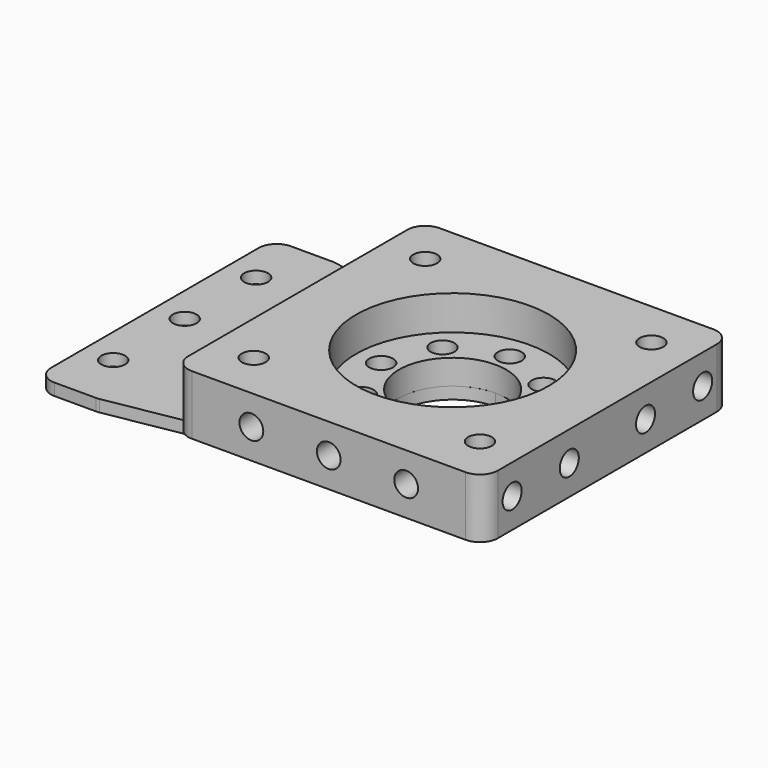
from build123d import *

# Parameters (mm, degrees)
F0_W             = 26
F0_H             = 26
F0_R             = 1
F0_R_2           = 4.5
F1_DEPTH         = 5
F2_R             = 1
F3_DEPTH         = 2
F4_R             = 8.1
F5_DEPTH         = 2.9
F6_R             = 1
F7_DEPTH         = 2
F8_R             = 1.5
F9_R             = 1
F10_DEPTH        = 5
F11_R            = 1
F12_DEPTH        = 1
F14_DEPTH        = 1
F15_R            = 1.5
F16_R            = 1
F17_DEPTH        = 4
F17_COPIES_COUNT = 2
F17_COPIES_PITCH = 22


# Not quite as in the source:
# - a pattern or mirror of a feature is missing from the dataset's text; its kind, count and spacing are read off the source's solid


with BuildPart() as f1:
    # F0 (on Top) → F1 (new body)
    with BuildSketch(Plane.XY):
        Rectangle(F0_W, F0_H)
        with Locations((-4.2426406871, -4.2426406871)):
            Circle(F0_R, mode=Mode.SUBTRACT)
        with Locations((0, -6)):
            Circle(F0_R, mode=Mode.SUBTRACT)
        with Locations((4.2426406871, -4.2426406871)):
            Circle(F0_R, mode=Mode.SUBTRACT)
        with Locations((-6, 0)):
            Circle(F0_R, mode=Mode.SUBTRACT)
        with Locations((-4.2426406871, 4.2426406871)):
            Circle(F0_R, mode=Mode.SUBTRACT)
        Circle(F0_R_2, mode=Mode.SUBTRACT)
        with Locations((6, 0)):
            Circle(F0_R, mode=Mode.SUBTRACT)
        with Locations((0, 6)):
            Circle(F0_R, mode=Mode.SUBTRACT)
        with Locations((4.2426406871, 4.2426406871)):
            Circle(F0_R, mode=Mode.SUBTRACT)
    extrude(amount=F1_DEPTH)

    # F2 (on face) → F3 (cut)
    with BuildSketch(Plane.XZ.offset(13)):
        with Locations((0, 2.5)):
            Circle(F2_R)
        with Locations((-6.5, 2.5)):
            Circle(F2_R)
        with Locations((6.5, 2.5)):
            Circle(F2_R)
    extrude(amount=-F3_DEPTH, mode=Mode.SUBTRACT)

    # F4 (on face) → F5 (cut)
    with BuildSketch(Plane.XY.offset(5)):
        Circle(F4_R)
    extrude(amount=-F5_DEPTH, mode=Mode.SUBTRACT)

    # F6 (on face) → F7 (cut)
    with BuildSketch(Plane(origin=(0, 13, 0), x_dir=(-1, 0, 0), z_dir=(0, 1, 0))):
        with Locations((6.5, 2.5)):
            Circle(F6_R)
        with Locations((0, 2.5)):
            Circle(F6_R)
        with Locations((-6.5, 2.5)):
            Circle(F6_R)
    extrude(amount=-F7_DEPTH, mode=Mode.SUBTRACT)

    # F8
    f8_edges = [f1.edges().sort_by_distance(p)[0] for p in [
        (-13, -13, 2.5),
        (13, -13, 2.5),
        (-13, 13, 2.5),
        (13, 13, 2.5),
    ]]
    fillet(f8_edges, radius=F8_R)

    # F9 (on face) → F10 (cut, through all)
    with BuildSketch(Plane.XY.offset(5)):
        with Locations((-9.5, 9)):
            Circle(F9_R)
        with Locations((9.5, 9)):
            Circle(F9_R)
        with Locations((-9.5, -9)):
            Circle(F9_R)
        with Locations((9.5, -9)):
            Circle(F9_R)
    extrude(amount=-F10_DEPTH, mode=Mode.SUBTRACT)

    # F16 (on face) → F17 (cut)
    with BuildSketch(Plane.YZ.offset(13)):
        with Locations((-4, 2.5)):
            Circle(F16_R)
        with Locations((-10, 2.5)):
            Circle(F16_R)
        with Locations((4, 2.5)):
            Circle(F16_R)
        with Locations((10, 2.5)):
            Circle(F16_R)
    f17 = extrude(amount=-F17_DEPTH, mode=Mode.SUBTRACT)

    # F17_copies: F17 ×2
    with Locations(*[(-i * F17_COPIES_PITCH, 0, 0) for i in range(1, F17_COPIES_COUNT)]):
        add(f17, mode=Mode.SUBTRACT)


with BuildPart() as f12:
    # F11 (on face) → F12 (new body)
    with BuildSketch(Plane(origin=(0, 0, 0), x_dir=(1, 0, 0), z_dir=(0, 0, -1))):
        with BuildLine():
            ThreePointArc((0, -4.5), (-4.5, 0), (0, 4.5))
            Line((0, 4.5), (2.5, 4.5))
            Line((2.5, 4.5), (2.5, 12.4))
            Line((2.5, 12.4), (-12.7, 12.4))
            ThreePointArc((-12.7, 12.4), (-12.9230249471, 11.974341649), (-13, 11.5))
            Line((-13, 11.5), (-13, -11.5))
            ThreePointArc((-13, -11.5), (-12.9230249471, -11.974341649), (-12.7, -12.4))
            Line((-12.7, -12.4), (2.5, -12.4))
            Line((2.5, -12.4), (2.5, -4.5))
            Line((2.5, -4.5), (0, -4.5))
        make_face()
        with Locations((-9.5, -9)):
            Circle(F11_R, mode=Mode.SUBTRACT)
        with Locations((-4.2426406871, -4.2426406871)):
            Circle(F11_R, mode=Mode.SUBTRACT)
        with Locations((0, -6)):
            Circle(F11_R, mode=Mode.SUBTRACT)
        with Locations((-9.5, 9)):
            Circle(F11_R, mode=Mode.SUBTRACT)
        with Locations((-6, 0)):
            Circle(F11_R, mode=Mode.SUBTRACT)
        with Locations((-4.2426406871, 4.2426406871)):
            Circle(F11_R, mode=Mode.SUBTRACT)
        with Locations((0, 6)):
            Circle(F11_R, mode=Mode.SUBTRACT)
        with BuildLine():
            ThreePointArc((-13, 11.5), (-12.9230249471, 11.974341649), (-12.7, 12.4))
            Line((-12.7, 12.4), (-25, 12.4))
            Line((-25, 12.4), (-25, -12.4))
            Line((-25, -12.4), (-12.7, -12.4))
            ThreePointArc((-12.7, -12.4), (-12.9230249471, -11.974341649), (-13, -11.5))
            Line((-13, -11.5), (-13, 11.5))
        make_face()
        with Locations((-22.5, -7.5)):
            Circle(F11_R, mode=Mode.SUBTRACT)
        with Locations((-22.5, 0)):
            Circle(F11_R, mode=Mode.SUBTRACT)
        with Locations((-22.5, 7.5)):
            Circle(F11_R, mode=Mode.SUBTRACT)
        with Locations((-9.5, 9)):
            Circle(F11_R)
        with Locations((-9.5, -9)):
            Circle(F11_R)
    extrude(amount=F12_DEPTH)

    # F13 (on face) → F14 (cut, through all)
    with BuildSketch(Plane(origin=(0, 0, -1), x_dir=(1, 0, 0), z_dir=(0, 0, -1))):
        Polygon((-19.9, 12.4), (2.5, 8.45), (2.5, 12.4), align=None)
        Polygon((-19.9, -12.4), (2.5, -12.4), (2.5, -8.45), align=None)
    extrude(amount=-F14_DEPTH, mode=Mode.SUBTRACT)

    # F15
    f15_edges = [f12.edges().sort_by_distance(p)[0] for p in [
        (2.5, -8.45, -0.5),
        (-19.9, -12.4, -0.5),
        (-25, -12.4, -0.5),
        (2.5, 4.5, -0.5),
        (2.5, -4.5, -0.5),
        (2.5, 8.45, -0.5),
        (-19.9, 12.4, -0.5),
        (-25, 12.4, -0.5),
    ]]
    fillet(f15_edges, radius=F15_R)


solid = Compound([f1.part, f12.part])
